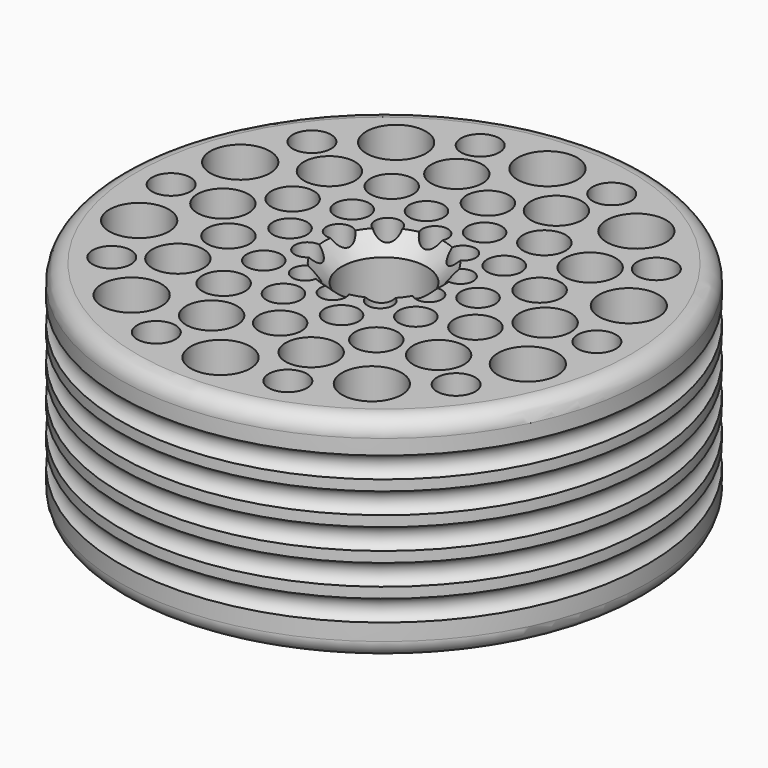
from build123d import *

# Parameters (mm, degrees)
F0_R     = 31
F0_R_2   = 2.25
F0_R_3   = 3.5
F0_R_4   = 3
F0_R_5   = 2.5
F0_R_6   = 2
F0_R_7   = 1.5
F0_R_8   = 5
F1_DEPTH = 12.5
F2_R     = 2
F3_R     = 1.4012473902


# Not quite as in the source:
# - a fillet or chamfer that OpenCascade refuses, or shapes differently, is made with other operations: its cross-section is extruded or revolved along the edge and cut away or added


with BuildPart() as f1:
    # F0 (on Top) → F1 (new body, symmetric)
    with BuildSketch(Plane.XY):
        Circle(F0_R)
        with Locations((-7.7254248594, -23.7764129074)):
            Circle(F0_R_2, mode=Mode.SUBTRACT)
        with Locations((-14.106846055, -19.416407865)):
            Circle(F0_R_3, mode=Mode.SUBTRACT)
        with Locations((-5.8485545322, -18)):
            Circle(F0_R_4, mode=Mode.SUBTRACT)
        with Locations((-20.2254248594, -14.6946313073)):
            Circle(F0_R_2, mode=Mode.SUBTRACT)
        with Locations((-22.8253563911, -7.416407865)):
            Circle(F0_R_3, mode=Mode.SUBTRACT)
        with Locations((-8.9637250975, -12.3375091642)):
            Circle(F0_R_5, mode=Mode.SUBTRACT)
        with Locations((-15.3117145503, -11.1246117975)):
            Circle(F0_R_4, mode=Mode.SUBTRACT)
        with Locations((-3.4116568104, -10.5)):
            Circle(F0_R_6, mode=Mode.SUBTRACT)
        with Locations((-14.5036118735, -4.7125091642)):
            Circle(F0_R_5, mode=Mode.SUBTRACT)
        with Locations((-8.9318334877, -6.4893568819)):
            Circle(F0_R_6, mode=Mode.SUBTRACT)
        with Locations((-4.4083893922, -6.0676274578)):
            Circle(F0_R_7, mode=Mode.SUBTRACT)
        with Locations((-7.1329238722, -2.3176274578)):
            Circle(F0_R_7, mode=Mode.SUBTRACT)
        with Locations((0, -24)):
            Circle(F0_R_3, mode=Mode.SUBTRACT)
        with Locations((7.7254248594, -23.7764129074)):
            Circle(F0_R_2, mode=Mode.SUBTRACT)
        with Locations((5.8485545322, -18)):
            Circle(F0_R_4, mode=Mode.SUBTRACT)
        with Locations((14.106846055, -19.416407865)):
            Circle(F0_R_3, mode=Mode.SUBTRACT)
        with Locations((0, -15.25)):
            Circle(F0_R_5, mode=Mode.SUBTRACT)
        with Locations((3.4116568104, -10.5)):
            Circle(F0_R_6, mode=Mode.SUBTRACT)
        with Locations((8.9637250975, -12.3375091642)):
            Circle(F0_R_5, mode=Mode.SUBTRACT)
        with Locations((15.3117145503, -11.1246117975)):
            Circle(F0_R_4, mode=Mode.SUBTRACT)
        with Locations((0, -7.5)):
            Circle(F0_R_7, mode=Mode.SUBTRACT)
        with Locations((4.4083893922, -6.0676274578)):
            Circle(F0_R_7, mode=Mode.SUBTRACT)
        with Locations((7.1329238722, -2.3176274578)):
            Circle(F0_R_7, mode=Mode.SUBTRACT)
        with Locations((8.9318334877, -6.4893568819)):
            Circle(F0_R_6, mode=Mode.SUBTRACT)
        with Locations((14.5036118735, -4.7125091642)):
            Circle(F0_R_5, mode=Mode.SUBTRACT)
        with Locations((20.2254248594, -14.6946313073)):
            Circle(F0_R_2, mode=Mode.SUBTRACT)
        with Locations((22.8253563911, -7.416407865)):
            Circle(F0_R_3, mode=Mode.SUBTRACT)
        with Locations((-25, 0)):
            Circle(F0_R_2, mode=Mode.SUBTRACT)
        with Locations((-18.9263200363, 0)):
            Circle(F0_R_4, mode=Mode.SUBTRACT)
        with Locations((-22.8253563911, 7.416407865)):
            Circle(F0_R_3, mode=Mode.SUBTRACT)
        with Locations((-20.2254248594, 14.6946313073)):
            Circle(F0_R_2, mode=Mode.SUBTRACT)
        with Locations((-11.0403533545, 0)):
            Circle(F0_R_6, mode=Mode.SUBTRACT)
        with Locations((-14.5036118735, 4.7125091642)):
            Circle(F0_R_5, mode=Mode.SUBTRACT)
        with Locations((-8.9318334877, 6.4893568819)):
            Circle(F0_R_6, mode=Mode.SUBTRACT)
        with Locations((-7.1329238722, 2.3176274578)):
            Circle(F0_R_7, mode=Mode.SUBTRACT)
        with Locations((-4.4083893922, 6.0676274578)):
            Circle(F0_R_7, mode=Mode.SUBTRACT)
        with Locations((-15.3117145503, 11.1246117975)):
            Circle(F0_R_4, mode=Mode.SUBTRACT)
        with Locations((-8.9637250975, 12.3375091642)):
            Circle(F0_R_5, mode=Mode.SUBTRACT)
        with Locations((-3.4116568104, 10.5)):
            Circle(F0_R_6, mode=Mode.SUBTRACT)
        with Locations((-14.106846055, 19.416407865)):
            Circle(F0_R_3, mode=Mode.SUBTRACT)
        with Locations((-5.8485545322, 18)):
            Circle(F0_R_4, mode=Mode.SUBTRACT)
        with Locations((-7.7254248594, 23.7764129074)):
            Circle(F0_R_2, mode=Mode.SUBTRACT)
        Circle(F0_R_8, mode=Mode.SUBTRACT)
        with Locations((7.1329238722, 2.3176274578)):
            Circle(F0_R_7, mode=Mode.SUBTRACT)
        with Locations((0, 7.5)):
            Circle(F0_R_7, mode=Mode.SUBTRACT)
        with Locations((4.4083893922, 6.0676274578)):
            Circle(F0_R_7, mode=Mode.SUBTRACT)
        with Locations((11.0403533545, 0)):
            Circle(F0_R_6, mode=Mode.SUBTRACT)
        with Locations((8.9318334877, 6.4893568819)):
            Circle(F0_R_6, mode=Mode.SUBTRACT)
        with Locations((14.5036118735, 4.7125091642)):
            Circle(F0_R_5, mode=Mode.SUBTRACT)
        with Locations((3.4116568104, 10.5)):
            Circle(F0_R_6, mode=Mode.SUBTRACT)
        with Locations((0, 15.25)):
            Circle(F0_R_5, mode=Mode.SUBTRACT)
        with Locations((15.3117145503, 11.1246117975)):
            Circle(F0_R_4, mode=Mode.SUBTRACT)
        with Locations((8.9637250975, 12.3375091642)):
            Circle(F0_R_5, mode=Mode.SUBTRACT)
        with Locations((18.9263200363, 0)):
            Circle(F0_R_4, mode=Mode.SUBTRACT)
        with Locations((22.8253563911, 7.416407865)):
            Circle(F0_R_3, mode=Mode.SUBTRACT)
        with Locations((25, 0)):
            Circle(F0_R_2, mode=Mode.SUBTRACT)
        with Locations((20.2254248594, 14.6946313073)):
            Circle(F0_R_2, mode=Mode.SUBTRACT)
        with Locations((5.8485545322, 18)):
            Circle(F0_R_4, mode=Mode.SUBTRACT)
        with Locations((14.106846055, 19.416407865)):
            Circle(F0_R_3, mode=Mode.SUBTRACT)
        with Locations((0, 24)):
            Circle(F0_R_3, mode=Mode.SUBTRACT)
        with Locations((7.7254248594, 23.7764129074)):
            Circle(F0_R_2, mode=Mode.SUBTRACT)
    extrude(amount=F1_DEPTH, both=True)

    # F2
    f2_edges = [f1.edges().sort_by_distance(p)[0] for p in [
        (-31, 0, 12.5),
        (-31, 0, -12.5),
    ]]
    fillet(f2_edges, radius=F2_R)

    # F3 (on Right) → F4 (revolve, cut)
    with BuildSketch(Plane.YZ):
        with Locations((31.6685475409, 3.8)):
            Circle(F3_R)
        with Locations((31.6685475409, 7.5)):
            Circle(F3_R)
        with Locations((31.6685475409, -7.3)):
            Circle(F3_R)
        with Locations((31.6685475409, -3.6)):
            Circle(F3_R)
        with Locations((31.6685475409, 0.1)):
            Circle(F3_R)
    revolve(axis=Axis((0, 0, -3.5231631172), (0, 0, -1)), mode=Mode.SUBTRACT)

    # F5: chamfer of 2 on 2 edges, made by hand

    # F5_s1 → F5_t2 (revolve, cut)
    with BuildSketch(Plane.XZ):
        Polygon((5, 10.5), (7, 12.5), (5, 12.5), align=None)
    revolve(axis=Axis((0, 0, 12.5), (0, 0, 1)), mode=Mode.SUBTRACT)

    # F5_s3 → F5_t4 (revolve, cut)
    with BuildSketch(Plane.XZ):
        Polygon((7, -12.5), (5, -10.5), (5, -12.5), align=None)
    revolve(axis=Axis((0, 0, -12.5), (0, 0, 1)), mode=Mode.SUBTRACT)


solid = f1.part
